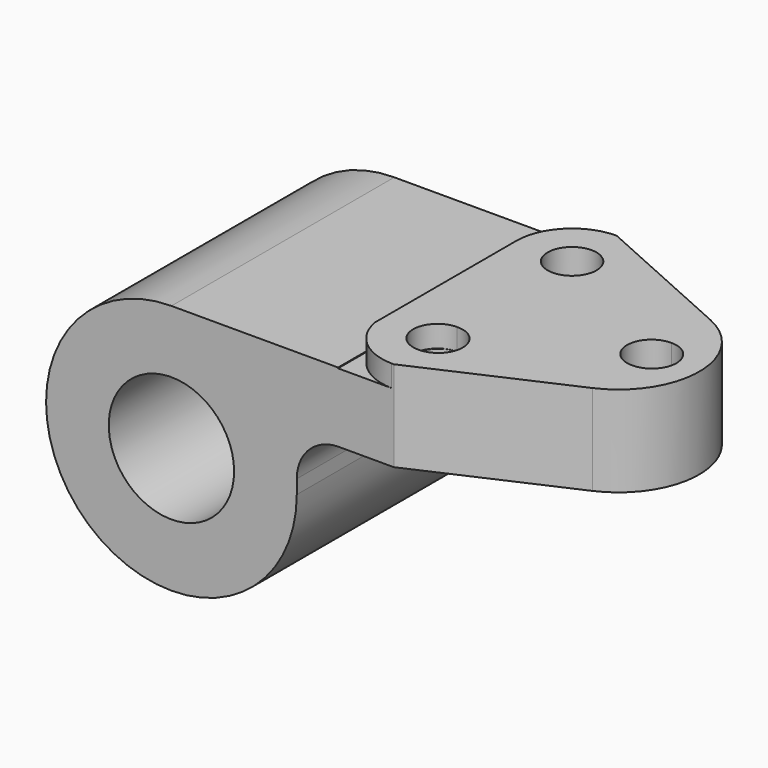
from build123d import *

# Parameters (mm, degrees)
F0_R     = 14.2875
F1_DEPTH = 63.5
F3_START = 28.40385
F2_R     = 5.5626
F3_DEPTH = 4.94635
F4_R     = 5.5626
F5_DEPTH = 33.3512


with BuildPart() as f1:
    # F0 (on Front) → F1 (new body)
    with BuildSketch(Plane.XZ):
        with BuildLine():
            Line((37.9924699664, 28.575), (0, 28.575))
            ThreePointArc((0, 28.575), (-20.2055762724, -20.2055762724), (28.575, 0))
            Line((28.575, 0), (28.575, 3.175))
            ThreePointArc((28.575, 3.175), (31.3648079092, 9.9101920908), (38.1, 12.7))
            Line((38.1, 12.7), (69.85, 12.7))
            Line((69.85, 12.7), (95.0348461551, 12.7))
            Line((95.0348461551, 12.7), (95.0348461551, 33.3502))
            Line((95.0348461551, 33.3502), (37.9924699664, 33.3502))
            Line((37.9924699664, 33.3502), (37.9924699664, 28.575))
        make_face()
        Circle(F0_R, mode=Mode.SUBTRACT)
    extrude(amount=F1_DEPTH)

    # F2 (on Top) → F3 (cut)
    with BuildSketch(Plane.XY.offset(F3_START)):
        with BuildLine():
            ThreePointArc((37.9924699664, -12.7), (41.6741160957, -3.757548703), (50.5849399165, 0))
            Line((50.5849399165, 0), (37.9924699664, 0))
            Line((37.9924699664, 0), (37.9924699664, -12.7))
        make_face()
        with BuildLine():
            Line((50.5849399165, 0), (50.8, 0))
            ThreePointArc((50.8, 0), (50.6924699583, 0.000455233), (50.5849399165, 0))
        make_face()
        with BuildLine():
            Line((37.9924699664, -63.5), (50.2103307418, -63.5))
            ThreePointArc((50.2103307418, -63.5), (42.2169815898, -60.4261048405), (37.9924699664, -52.9765435338))
            Line((37.9924699664, -52.9765435338), (37.9924699664, -63.5))
        make_face()
        with BuildLine():
            ThreePointArc((50.2103307418, -63.5), (50.5051653709, -63.5034228021), (50.8, -63.5))
            Line((50.8, -63.5), (50.2103307418, -63.5))
        make_face()
        with Locations((84.1502, -31.75)):
            Circle(F2_R)
        with Locations((50.6924699583, -12.699544767)):
            Circle(F2_R)
        with Locations((50.5051653709, -50.8034228021)):
            Circle(F2_R)
    extrude(amount=F3_DEPTH, mode=Mode.SUBTRACT)

    # F4 (on Top) → F5 (cut, through all)
    with BuildSketch(Plane.XY):
        with BuildLine():
            Line((84.0428003407, -48.5551651302), (50.6926003407, -63.5))
            Line((50.6926003407, -63.5), (95.0348461551, -63.5))
            Line((95.0348461551, -63.5), (95.0348461551, 0))
            Line((95.0348461551, 0), (50.6926003407, 0.0004552323))
            Line((50.6926003407, 0.0004552323), (84.0428003407, -14.9443796375))
            ThreePointArc((84.0428003407, -14.9443796375), (94.9275939219, -31.7497723839), (84.0428003407, -48.5551651302))
        make_face()
        with Locations((84.0428003407, -31.7497723839)):
            Circle(F4_R)
        with Locations((50.6924699583, -12.699544767)):
            Circle(F4_R)
        with Locations((50.6926003407, -50.8)):
            Circle(F4_R)
    extrude(amount=F5_DEPTH, mode=Mode.SUBTRACT)


solid = f1.part
